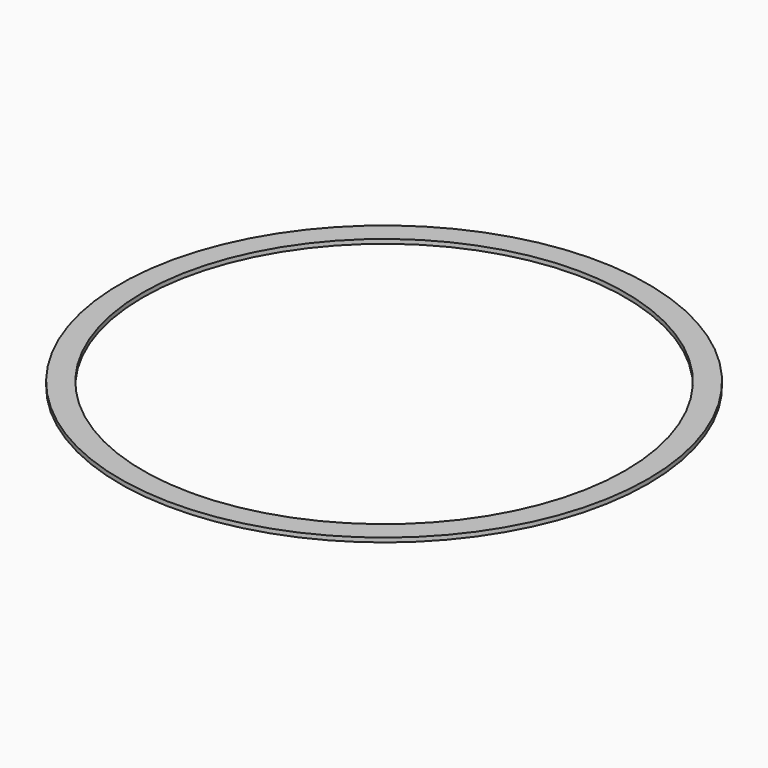
from build123d import *

# Parameters (mm, degrees)
F0_R     = 293.93007
F0_R_2   = 268.53007
F1_DEPTH = 4.7625


# Not quite as in the source:
# - a length typed as a fraction of an inch, garbled in the dataset ("3 / 203.2 mm" for 3/8 in), is restored


with BuildPart() as f1:
    # F0 (on Top) → F1 (new body)
    with BuildSketch(Plane.XY):
        Circle(F0_R)
        Circle(F0_R_2, mode=Mode.SUBTRACT)
    extrude(amount=F1_DEPTH)


solid = f1.part
